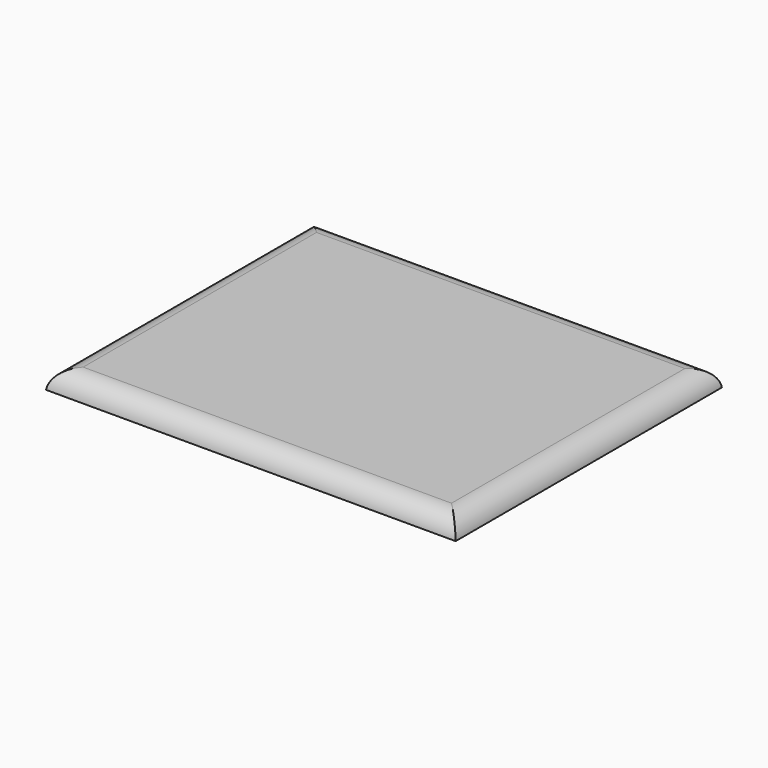
from build123d import *

# Parameters (mm, degrees)
F0_W        = 100.4
F0_H        = 81.6
F1_DEPTH    = 4.5
F2_T1_DEPTH = 125.6339057619
F2_T3_DEPTH = 106.8339057619
F3_T        = -2.54


# Not quite as in the source:
# - a fillet or chamfer that OpenCascade refuses, or shapes differently, is made with other operations: its cross-section is extruded or revolved along the edge and cut away or added


with BuildPart() as f1:
    # F0 (on Top) → F1 (new body)
    with BuildSketch(Plane.XY):
        with Locations((-0.9694248438, 10.5918823534)):
            Rectangle(F0_W, F0_H)
    extrude(amount=F1_DEPTH)

    # F2: fillet of radius 5.08 on 4 edges, made by hand

    # F2_s2 → F2_t1 (cut)
    with BuildSketch(Plane.YZ.offset(-63.7863777247)):
        with BuildLine():
            ThreePointArc((51.3918823534, 0), (49.7259295019, 3.2116223441), (46.345101201, 4.5))
            Line((46.345101201, 4.5), (51.3918823534, 4.5))
            Line((51.3918823534, 4.5), (51.3918823534, 0))
        make_face()
        with BuildLine():
            ThreePointArc((-30.2081176466, 0), (-28.5421647951, 3.2116223441), (-25.1613364942, 4.5))
            Line((-25.1613364942, 4.5), (-30.2081176466, 4.5))
            Line((-30.2081176466, 4.5), (-30.2081176466, 0))
        make_face()
    extrude(amount=F2_T1_DEPTH, mode=Mode.SUBTRACT)

    # F2_s4 → F2_t3 (cut)
    with BuildSketch(Plane.XZ.offset(-64.0088352343)):
        with BuildLine():
            ThreePointArc((-51.1694248438, 0), (-49.5034719923, 3.2116223441), (-46.1226436914, 4.5))
            Line((-46.1226436914, 4.5), (-51.1694248438, 4.5))
            Line((-51.1694248438, 4.5), (-51.1694248438, 0))
        make_face()
        with BuildLine():
            ThreePointArc((49.2305751562, 0), (47.5646223047, 3.2116223441), (44.1837940038, 4.5))
            Line((44.1837940038, 4.5), (49.2305751562, 4.5))
            Line((49.2305751562, 4.5), (49.2305751562, 0))
        make_face()
    extrude(amount=F2_T3_DEPTH, mode=Mode.SUBTRACT)

    # F3
    f3_openings = [f1.faces().sort_by_distance(p)[0] for p in [
        (-0.969425, 10.591882, 0),
    ]]
    offset(amount=F3_T, openings=f3_openings)


solid = f1.part
